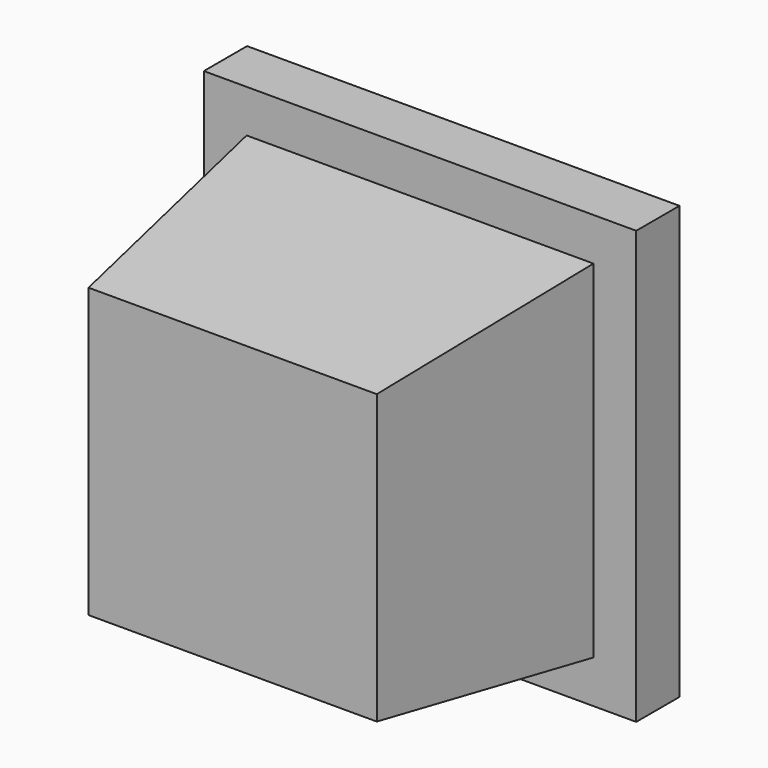
from build123d import *

# Parameters (mm, degrees)
F0_W         = 30.48
F0_H         = 30.48
F0_W_2       = 25.4
F0_H_2       = 25.4
F1_DEPTH     = 3.81
F0_W_3       = 15.24
F0_H_3       = 15.24
F2_DEPTH     = 20.32
F3_DEPTH     = 2.54
F4_T4_DEPTH  = 131.0338200082
F4_T9_DEPTH  = 131.0338200082
F4_T14_DEPTH = 131.0338200082
F4_T19_DEPTH = 131.0338200082


# Not quite as in the source:
# - a fillet or chamfer that OpenCascade refuses, or shapes differently, is made with other operations: its cross-section is extruded or revolved along the edge and cut away or added


with BuildPart() as f1:
    # F0 (on Front) → F1 (new body)
    with BuildSketch(Plane.XZ):
        Rectangle(F0_W, F0_H)
        Rectangle(F0_W_2, F0_H_2, mode=Mode.SUBTRACT)
    extrude(amount=F1_DEPTH)

    # F0 (on Front) → F2 (join)
    with BuildSketch(Plane.XZ):
        Rectangle(F0_W_2, F0_H_2)
        Rectangle(F0_W_3, F0_H_3, mode=Mode.SUBTRACT)
        Rectangle(F0_W_3, F0_H_3)
    extrude(amount=F2_DEPTH)

    # F0 (on Front) → F3 (cut)
    with BuildSketch(Plane.XZ):
        Rectangle(F0_W_2, F0_H_2)
        Rectangle(F0_W_3, F0_H_3, mode=Mode.SUBTRACT)
        Rectangle(F0_W_3, F0_H_3)
    extrude(amount=F3_DEPTH, mode=Mode.SUBTRACT)

    # F4: chamfer of 2.54 x 20.32 on 4 edges, made by hand


with BuildPart() as f4_tool2:
    # F4_s3 → F4_t4 (new body)
    with BuildSketch(Plane.YZ.offset(65.5169100041)):
        Polygon((0, 12.7), (-20.32, 10.16), (-20.32, 12.7), align=None)
    extrude(amount=-F4_T4_DEPTH)

    split(bisect_by=Plane.XZ.offset(3.81), keep=Keep.TOP)


with BuildPart() as f1_1:
    add(f1.part)

    # F4_t1: cut F4_tool2
    add(f4_tool2.part, mode=Mode.SUBTRACT)


with BuildPart() as f4_tool7:
    # F4_s8 → F4_t9 (new body)
    with BuildSketch(Plane.XY.offset(65.5169100041)):
        Polygon((-12.7, 0), (-10.16, -20.32), (-12.7, -20.32), align=None)
    extrude(amount=-F4_T9_DEPTH)

    split(bisect_by=Plane.XZ.offset(3.81), keep=Keep.TOP)


with BuildPart() as f1_2:
    add(f1_1.part)

    # F4_t6: cut F4_tool7
    add(f4_tool7.part, mode=Mode.SUBTRACT)


with BuildPart() as f4_tool12:
    # F4_s13 → F4_t14 (new body)
    with BuildSketch(Plane.YZ.offset(-65.5169100041)):
        Polygon((0, -12.7), (-20.32, -10.16), (-20.32, -12.7), align=None)
    extrude(amount=F4_T14_DEPTH)

    split(bisect_by=Plane.XZ.offset(3.81), keep=Keep.TOP)


with BuildPart() as f1_3:
    add(f1_2.part)

    # F4_t11: cut F4_tool12
    add(f4_tool12.part, mode=Mode.SUBTRACT)


with BuildPart() as f4_tool17:
    # F4_s18 → F4_t19 (new body)
    with BuildSketch(Plane.XY.offset(-65.5169100041)):
        Polygon((12.7, 0), (10.16, -20.32), (12.7, -20.32), align=None)
    extrude(amount=F4_T19_DEPTH)

    split(bisect_by=Plane.XZ.offset(3.81), keep=Keep.TOP)


with BuildPart() as f1_4:
    add(f1_3.part)

    # F4_t16: cut F4_tool17
    add(f4_tool17.part, mode=Mode.SUBTRACT)


solid = f1_4.part
